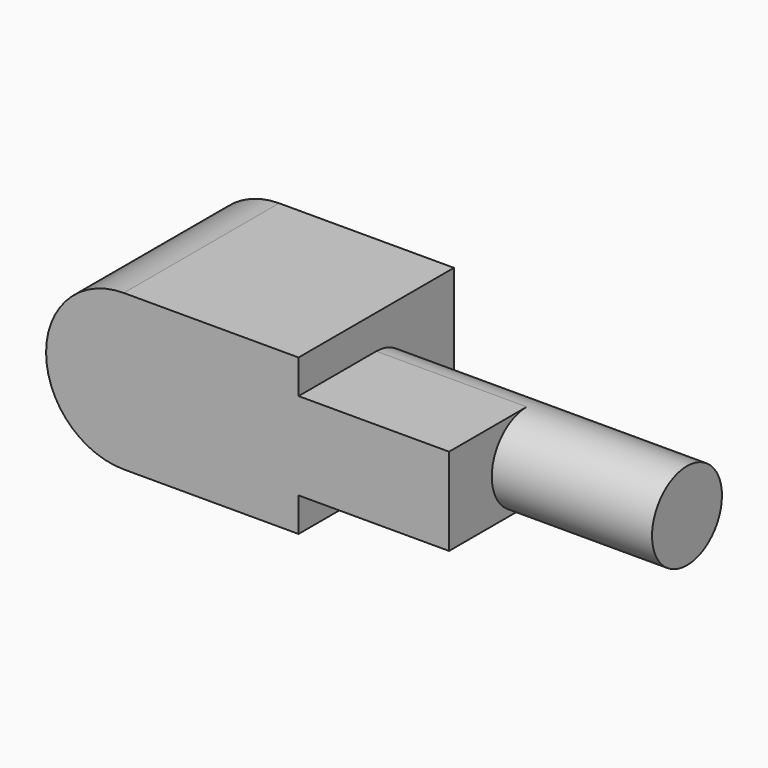
from build123d import *
from build123d import SkipClean  # not in build123d's __all__

# Parameters (mm, degrees)
F0_W     = 812.8
F0_H     = 457.2
F1_DEPTH = 1016
F3_DEPTH = 812.8
F4_DEPTH = 812.8
F5_DEPTH = 25.4


# Not quite as in the source:
# - a feature names something its author has since deleted; it is built from what else it names


with BuildPart() as f1:
    # F0 (on Front) → F1 (new body)
    with BuildSketch(Plane.XZ):
        with BuildLine():
            ThreePointArc((0, -406.4), (287.3681958742, -287.3681958742), (406.4, 0))
            ThreePointArc((406.4, 0), (287.3681958742, 287.3681958742), (0, 406.4))
            Line((0, 406.4), (0, -406.4))
        make_face()
        with BuildLine():
            ThreePointArc((0, 406.4), (287.3681958742, 287.3681958742), (406.4, 0))
            ThreePointArc((406.4, 0), (287.3681958742, -287.3681958742), (0, -406.4))
            Line((0, -406.4), (914.4, -406.4))
            Line((914.4, -406.4), (914.4, -228.6))
            Line((914.4, -228.6), (914.4, 228.6))
            Line((914.4, 228.6), (914.4, 406.4))
            Line((914.4, 406.4), (0, 406.4))
        make_face()
        with BuildLine():
            Line((0, -406.4), (0, 406.4))
            ThreePointArc((0, 406.4), (-406.4, 0), (0, -406.4))
        make_face()
        with Locations((1320.8, 0)):
            Rectangle(F0_W, F0_H)
    extrude(amount=F1_DEPTH)

    # F2 (on face) → F3 (cut)
    with BuildSketch(Plane.YZ.offset(1727.2)):
        with BuildLine():
            ThreePointArc((-508, 228.6), (-346.3553898207, 161.6446101792), (-279.4, 0))
            ThreePointArc((-279.4, 0), (-346.3553898207, -161.6446101792), (-508, -228.6))
            Line((-508, -228.6), (0, -228.6))
            Line((0, -228.6), (0, 228.6))
            Line((0, 228.6), (-508, 228.6))
        make_face()
    extrude(amount=-F3_DEPTH, mode=Mode.SUBTRACT)

    # F2 (on face) → F4 (join)
    with BuildSketch(Plane.YZ.offset(1727.2)):
        with BuildLine():
            ThreePointArc((-508, -228.6), (-346.3553898207, -161.6446101792), (-279.4, 0))
            ThreePointArc((-279.4, 0), (-346.3553898207, 161.6446101792), (-508, 228.6))
            ThreePointArc((-508, 228.6), (-736.6, 0), (-508, -228.6))
        make_face()
    with SkipClean():  # cleaning this boolean's faces spoils the solid; the shape is the same uncleaned
        extrude(amount=F4_DEPTH)

    # F2 (on face) → F5 (cut)
    with BuildSketch(Plane.YZ.offset(1727.2)):
        with BuildLine():
            ThreePointArc((-508, -228.6), (-736.6, 0), (-508, 228.6))
            Line((-508, 228.6), (-1016, 228.6))
            Line((-1016, 228.6), (-1016, -228.6))
            Line((-1016, -228.6), (-508, -228.6))
        make_face()
    extrude(amount=-F5_DEPTH, mode=Mode.SUBTRACT)


solid = f1.part
